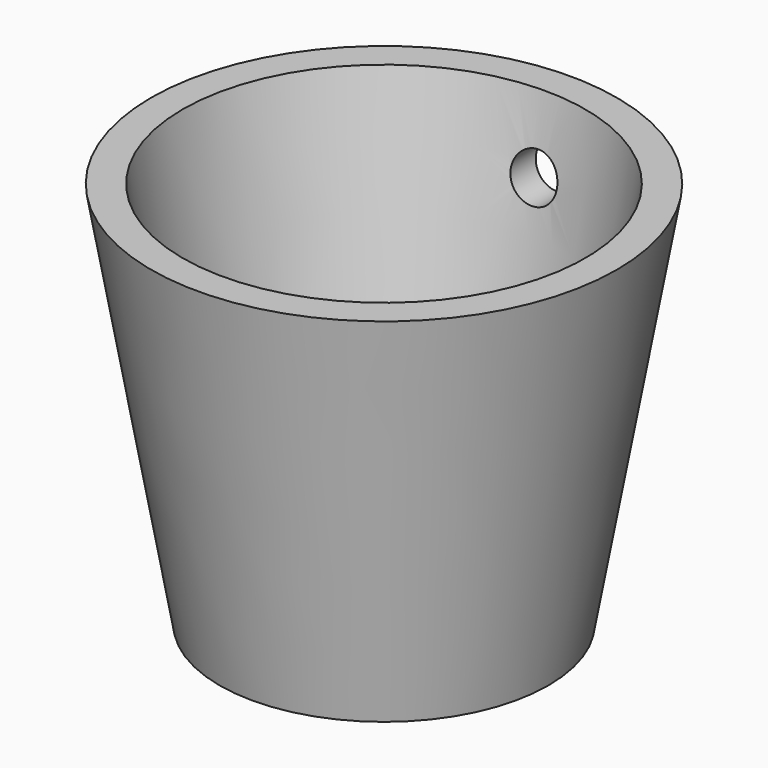
from build123d import *

# Parameters (mm, degrees)
F2_T     = -5.08
F3_R     = 3.81
F4_DEPTH = 304.8


# Not quite as in the source:
# - a feature names something its author has since deleted; it is built from what else it names


with BuildPart() as f1:
    # F0 (on Front) → F1 (revolve)
    with BuildSketch(Plane.XZ):
        Polygon((0, 0), (0, 63.5), (-38.1, 63.5), (-26.903236725, 0), align=None)
    revolve(axis=Axis((0, 0, 31.75), (0, 0, 1)))

    # F2
    f2_openings = [f1.faces().sort_by_distance(p)[0] for p in [
        (0, 0, 63.5),
    ]]
    offset(amount=F2_T, openings=f2_openings)

    # F3 (on Front) → F4 (cut)
    with BuildSketch(Plane.XZ):
        with Locations((0, 51.8186431976)):
            Circle(F3_R)
    extrude(amount=-F4_DEPTH, mode=Mode.SUBTRACT)


solid = f1.part
